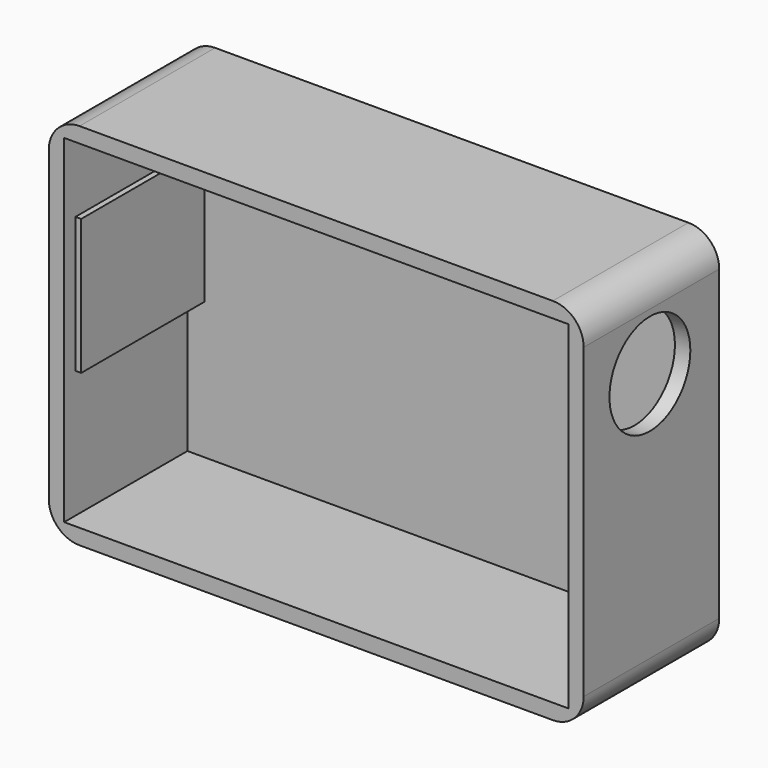
from build123d import *

# Parameters (mm, degrees)
F0_W        = 83.1117276102
F0_H        = 55.7723436505
F1_DEPTH    = 25.4
F2_T        = 2.54
F3_T1_DEPTH = 53.34
F5_D        = 16.66748
F5_DEPTH    = 56.4907174323
F6_W        = 0.9412951767
F6_H        = 22.3557362333
F7_DEPTH    = 25.4


# Not quite as in the source:
# - a fillet or chamfer that OpenCascade refuses, or shapes differently, is made with other operations: its cross-section is extruded or revolved along the edge and cut away or added


with BuildPart() as f1:
    # F0 (on Front) → F1 (new body)
    with BuildSketch(Plane.XZ):
        with Locations((12.3938536271, -8.5663376376)):
            Rectangle(F0_W, F0_H)
    extrude(amount=F1_DEPTH)

    # F2
    f2_openings = [f1.faces().sort_by_distance(p)[0] for p in [
        (12.393854, -25.4, -8.566338),
    ]]
    offset(amount=F2_T, openings=f2_openings, kind=Kind.INTERSECTION)

    # F3: fillet of radius 5.08 on 4 edges, made by hand

    # F3_s2 → F3_t1 (cut)
    with BuildSketch(Plane.XZ.offset(-15.24)):
        with BuildLine():
            ThreePointArc((51.4097174323, 21.8598341876), (55.0018198807, 20.3719366361), (56.4897174323, 16.7798341876))
            Line((56.4897174323, 16.7798341876), (56.4897174323, 21.8598341876))
            Line((56.4897174323, 21.8598341876), (51.4097174323, 21.8598341876))
        make_face()
        with BuildLine():
            ThreePointArc((-26.622010178, 21.8598341876), (-30.2141126264, 20.3719366361), (-31.702010178, 16.7798341876))
            Line((-31.702010178, 16.7798341876), (-31.702010178, 21.8598341876))
            Line((-31.702010178, 21.8598341876), (-26.622010178, 21.8598341876))
        make_face()
        with BuildLine():
            ThreePointArc((-31.702010178, -33.9125094628), (-30.2141126264, -37.5046119113), (-26.622010178, -38.9925094628))
            Line((-26.622010178, -38.9925094628), (-31.702010178, -38.9925094628))
            Line((-31.702010178, -38.9925094628), (-31.702010178, -33.9125094628))
        make_face()
        with BuildLine():
            ThreePointArc((51.4097174323, -38.9925094628), (55.0018198807, -37.5046119113), (56.4897174323, -33.9125094628))
            Line((56.4897174323, -33.9125094628), (56.4897174323, -38.9925094628))
            Line((56.4897174323, -38.9925094628), (51.4097174323, -38.9925094628))
        make_face()
    extrude(amount=F3_T1_DEPTH, mode=Mode.SUBTRACT)

    # F5 (through all, one way)
    with BuildSketch(Plane(origin=(0, 0, 0), x_dir=(0, 1, 0), z_dir=(-1, 0, 0))):
        with Locations((-11.7502789944, -7.3858899996)):
            Circle(F5_D / 2)
    extrude(amount=-F5_DEPTH, mode=Mode.SUBTRACT)

    # F6 (on Front) → F7 (join)
    with BuildSketch(Plane.XZ):
        with Locations((-26.8268827349, -2.7062208392)):
            Rectangle(F6_W, F6_H)
    extrude(amount=F7_DEPTH)


solid = f1.part
